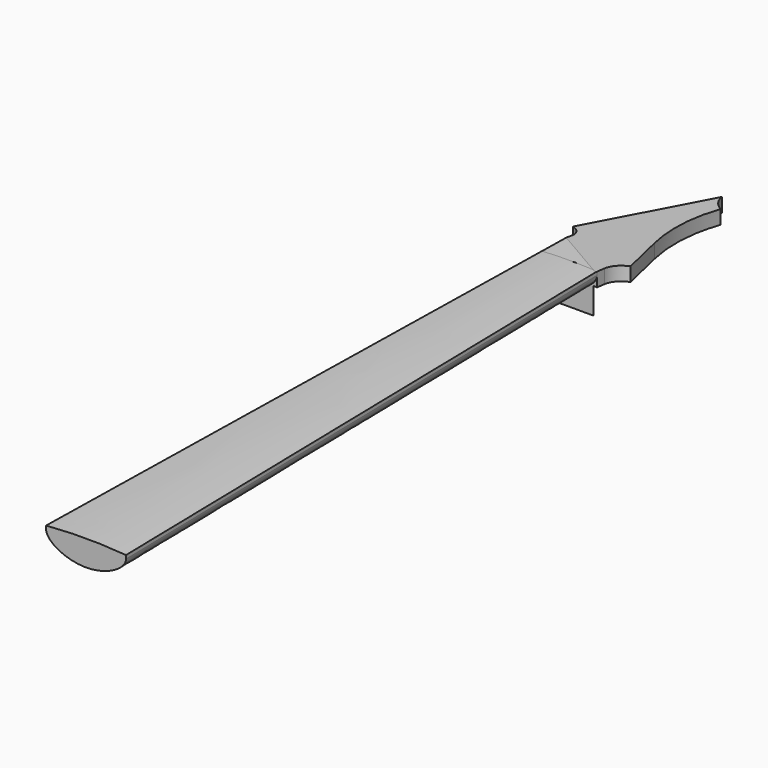
from build123d import *

# Parameters (mm, degrees)
F17_W          = 64.5110210379
F17_H          = 35
F18_DEPTH      = 165.0861956251
F21_DEPTH      = 300.8879553896
F21_DEPTH_BACK = 107.3482027968
F23_DEPTH      = 35.0010001


# Not quite as in the source:
# - ends of sketch curves that miss each other by under 0.0002 mm in the source are joined


with BuildPart() as f16:
    # F12 (on plane+point) → F16 section 0
    with BuildSketch(Plane.XZ.offset(-485.775)):
        with BuildLine():
            Line((24, -3), (24, 0))
            ThreePointArc((24, 0), (0, 0.6702898704), (-24, 0))
            Line((-24, 0), (-24, -3))
            add(Edge.make_bspline(
                [(0, -18.3297101296), (-8.1108585, -18.3297101296), (-24, -11.7364646867), (-24, -3)],
                knots=[0, 0, 0, 0, 28.4780619541, 28.4780619541, 28.4780619541, 28.4780619541], degree=3))
            add(Edge.make_bspline(
                [(0, -18.3297101296), (8.1108585, -18.3297101296), (24, -11.7364646867), (24, -3)],
                knots=[0, 0, 0, 0, 28.4780619541, 28.4780619541, 28.4780619541, 28.4780619541], degree=3))
        make_face()
    # F15 (on plane+point) → F16 section 1
    with BuildSketch(Plane.XZ.offset(41.2637528239)):
        with BuildLine():
            Line((34.849441672, -3), (34.849441672, 0))
            ThreePointArc((34.849441672, 0), (-4.636e-07, 1.414516756), (-34.849441672, 0))
            Line((-34.849441672, 0), (-34.849441672, -3))
            add(Edge.make_bspline(
                [(0, -20.8934800247), (-18.3918643743, -20.8934800247), (-34.849441672, -11.1013991282), (-34.849441672, -3)],
                knots=[0, 0, 0, 0, 39.1747394662, 39.1747394662, 39.1747394662, 39.1747394662], degree=3))
            add(Edge.make_bspline(
                [(0, -20.8934800247), (18.3918643743, -20.8934800247), (34.849441672, -11.1013991282), (34.849441672, -3)],
                knots=[0, 0, 0, 0, 39.1747394662, 39.1747394662, 39.1747394662, 39.1747394662], degree=3))
        make_face()
    loft()

    # F17 (on plane+point) → F18 (join, through all)
    with BuildSketch(Plane.XZ.offset(-485.775)):
        with Locations((0.3923069216, -17.5)):
            Rectangle(F17_W, F17_H)
    extrude(amount=-F18_DEPTH)

    # F20 (on line) → F21 (cut, two sides)
    with BuildSketch(Plane(origin=(-216.1177251342, 125.7026275723, 0), x_dir=(-0.5027782463, -0.8644154297, 0), z_dir=(-0.8644154297, 0.5027782463, 0))) as f21_sk:
        Polygon((-579.0290724854, -19.5657188317), (-430.4126832009, 0), (-430.4126832009, 11.4312007947), (-603.4596902493, 11.4312007947), (-603.4596902493, -22.782070678), align=None)
        Polygon((-577.4627581787, -31.4630571682), (-579.0290724854, -19.5657188317), (-603.4596902493, -22.782070678), (-603.4596902493, -42.47670056), (-430.4126832009, -42.47670056), (-430.4126832009, -12.103547527), align=None)
    extrude(amount=-F21_DEPTH, mode=Mode.SUBTRACT)
    extrude(f21_sk.sketch, amount=F21_DEPTH_BACK, mode=Mode.SUBTRACT)

    # F22 (on Top) → F23 (cut, through all)
    with BuildSketch(Plane.XY):
        with BuildLine():
            Line((-24, 485.775), (-23.4689132846, 511.5738649171))
            Line((-23.4689132846, 511.5738649171), (-23.3351348237, 518.0724881039))
            ThreePointArc((-23.3351348237, 518.0724881039), (-25.6339997847, 525.2791071894), (-31.8632035974, 529.5706289024))
            Line((-31.8632035974, 529.5706289024), (0.8434898226, 650.8611956251))
            ThreePointArc((0.8434898226, 650.8611956251), (5.0240250103, 641.5455786867), (12.5804428166, 634.6783999841))
            ThreePointArc((12.5804428166, 634.6783999841), (11.496048805, 594.1758564179), (19.2548236248, 554.408616647))
            Line((19.2548236248, 554.408616647), (32.6478174405, 511.4794017912))
            ThreePointArc((32.6478174405, 511.4794017912), (26.0643094519, 503.8032110141), (23.8319180476, 493.9400010445))
            Line((23.8319180476, 493.9400010445), (24.0377310644, 483.9421192188))
            Line((24.0377310644, 483.9421192188), (47.9396730661, 474.6490120888))
            Line((47.9396730661, 474.6490120888), (47.9396730661, 656.2497676849))
            Line((47.9396730661, 656.2497676849), (-50.3920817524, 656.2497676849))
            Line((-50.3920817524, 656.2497676849), (-50.3920817524, 480.0127209663))
            Line((-50.3920817524, 480.0127209663), (-24, 485.775))
        make_face()
    extrude(amount=-F23_DEPTH, mode=Mode.SUBTRACT)


solid = f16.part
